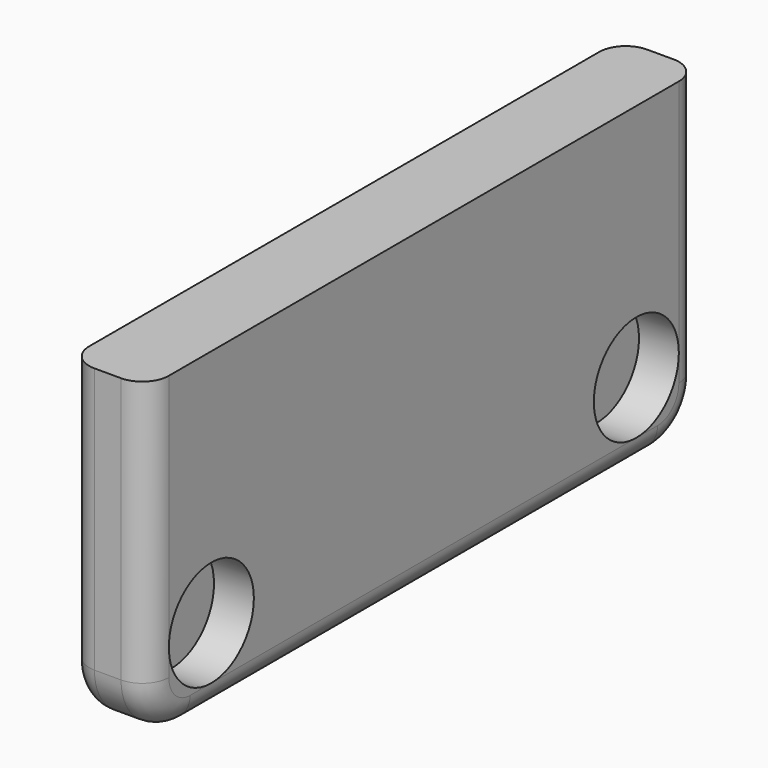
from build123d import *

# Parameters (mm, degrees)
F0_W     = 15
F0_H     = 130
F1_DEPTH = 60
F2_R     = 10
F3_DEPTH = 7.5
F4_R     = 10
F5_R     = 4.99999


# Not quite as in the source:
# - a fillet or chamfer is up to 0.001 mm smaller than in the source, because OpenCascade refuses the exact size


with BuildPart() as f1:
    # F0 (on Top) → F1 (new body)
    with BuildSketch(Plane.XY):
        Rectangle(F0_W, F0_H)
    extrude(amount=F1_DEPTH)

    # F2 (on face) → F3 (cut)
    with BuildSketch(Plane.YZ.offset(7.5)):
        with Locations((-50, 15)):
            Circle(F2_R)
        with Locations((50, 15)):
            Circle(F2_R)
    extrude(amount=-F3_DEPTH, mode=Mode.SUBTRACT)

    # F4
    f4_edges = [f1.edges().sort_by_distance(p)[0] for p in [
        (0, -65, 0),
        (0, 65, 0),
    ]]
    fillet(f4_edges, radius=F4_R)

    # F5 (radius 5 in the source; OpenCascade refuses exactly that, so slightly less here)
    f5_edges = [f1.edges().sort_by_distance(p)[0] for p in [
        (7.5, 0, 0),
        (-7.5, 0, 0),
    ]]
    fillet(f5_edges, radius=F5_R)


solid = f1.part
